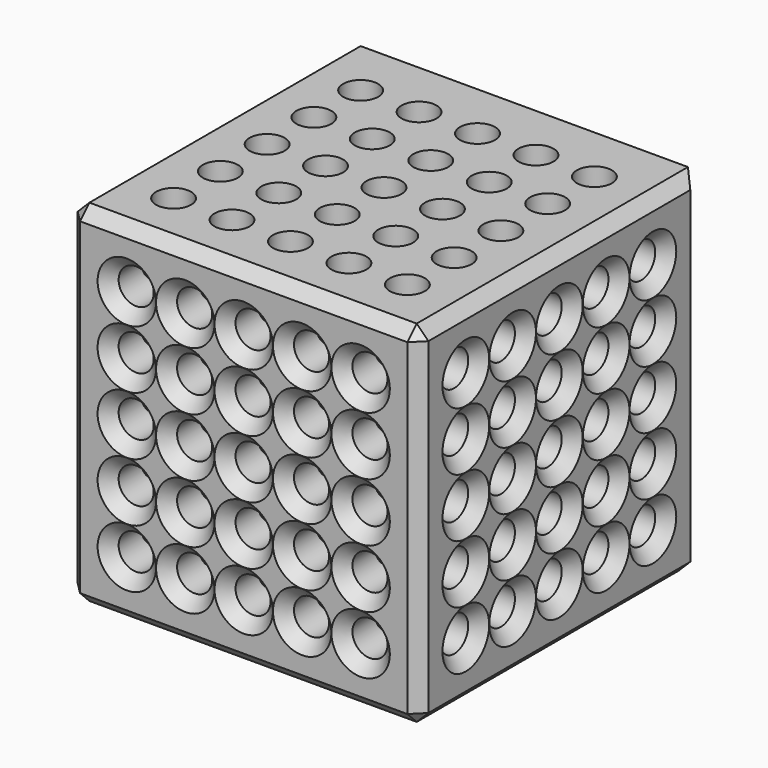
from build123d import *

# Parameters (mm, degrees)
F0_W     = 150
F0_H     = 150
F1_DEPTH = 150
F2_R     = 7.5
F3_DEPTH = 150.001
F4_R     = 7.5
F5_DEPTH = 150.001
F6_R     = 7.5
F7_DEPTH = 150.001
F8_SIZE  = 4.99999


# Not quite as in the source:
# - a fillet or chamfer is up to 0.001 mm smaller than in the source, because OpenCascade refuses the exact size


with BuildPart() as f1:
    # F0 (on Front) → F1 (new body)
    with BuildSketch(Plane.XZ):
        Rectangle(F0_W, F0_H)
    extrude(amount=F1_DEPTH)

    # F2 (on face) → F3 (cut, through all)
    with BuildSketch(Plane.XZ.offset(150)):
        with Locations((50, 50)):
            Circle(F2_R)
        with Locations((50, 25)):
            Circle(F2_R)
        with Locations((50, 0)):
            Circle(F2_R)
        with Locations((50, -25)):
            Circle(F2_R)
        with Locations((50, -50)):
            Circle(F2_R)
        with Locations((25, 50)):
            Circle(F2_R)
        with Locations((25, 25)):
            Circle(F2_R)
        with Locations((25, 0)):
            Circle(F2_R)
        with Locations((25, -25)):
            Circle(F2_R)
        with Locations((25, -50)):
            Circle(F2_R)
        with Locations((0, 50)):
            Circle(F2_R)
        with Locations((0, 25)):
            Circle(F2_R)
        Circle(F2_R)
        with Locations((0, -25)):
            Circle(F2_R)
        with Locations((0, -50)):
            Circle(F2_R)
        with Locations((-25, 50)):
            Circle(F2_R)
        with Locations((-25, 25)):
            Circle(F2_R)
        with Locations((-25, 0)):
            Circle(F2_R)
        with Locations((-25, -25)):
            Circle(F2_R)
        with Locations((-25, -50)):
            Circle(F2_R)
        with Locations((-50, 50)):
            Circle(F2_R)
        with Locations((-50, 25)):
            Circle(F2_R)
        with Locations((-50, 0)):
            Circle(F2_R)
        with Locations((-50, -25)):
            Circle(F2_R)
        with Locations((-50, -50)):
            Circle(F2_R)
    extrude(amount=-F3_DEPTH, mode=Mode.SUBTRACT)

    # F4 (on face) → F5 (cut, through all)
    with BuildSketch(Plane.YZ.offset(75)):
        with Locations((-25, 50)):
            Circle(F4_R)
        with Locations((-25, 25)):
            Circle(F4_R)
        with Locations((-25, 0)):
            Circle(F4_R)
        with Locations((-25, -25)):
            Circle(F4_R)
        with Locations((-25, -50)):
            Circle(F4_R)
        with Locations((-50, 50)):
            Circle(F4_R)
        with Locations((-50, 25)):
            Circle(F4_R)
        with Locations((-50, 0)):
            Circle(F4_R)
        with Locations((-50, -25)):
            Circle(F4_R)
        with Locations((-50, -50)):
            Circle(F4_R)
        with Locations((-75, 50)):
            Circle(F4_R)
        with Locations((-75, 25)):
            Circle(F4_R)
        with Locations((-75, 0)):
            Circle(F4_R)
        with Locations((-75, -25)):
            Circle(F4_R)
        with Locations((-75, -50)):
            Circle(F4_R)
        with Locations((-100, 50)):
            Circle(F4_R)
        with Locations((-100, 25)):
            Circle(F4_R)
        with Locations((-100, 0)):
            Circle(F4_R)
        with Locations((-100, -25)):
            Circle(F4_R)
        with Locations((-100, -50)):
            Circle(F4_R)
        with Locations((-125, 50)):
            Circle(F4_R)
        with Locations((-125, 25)):
            Circle(F4_R)
        with Locations((-125, 0)):
            Circle(F4_R)
        with Locations((-125, -25)):
            Circle(F4_R)
        with Locations((-125, -50)):
            Circle(F4_R)
    extrude(amount=-F5_DEPTH, mode=Mode.SUBTRACT)

    # F6 (on face) → F7 (cut, through all)
    with BuildSketch(Plane(origin=(0, 0, -75), x_dir=(1, 0, 0), z_dir=(0, 0, -1))):
        with Locations((50, 125)):
            Circle(F6_R)
        with Locations((50, 100)):
            Circle(F6_R)
        with Locations((50, 75)):
            Circle(F6_R)
        with Locations((50, 50)):
            Circle(F6_R)
        with Locations((50, 25)):
            Circle(F6_R)
        with Locations((25, 125)):
            Circle(F6_R)
        with Locations((25, 100)):
            Circle(F6_R)
        with Locations((25, 75)):
            Circle(F6_R)
        with Locations((25, 50)):
            Circle(F6_R)
        with Locations((25, 25)):
            Circle(F6_R)
        with Locations((0, 125)):
            Circle(F6_R)
        with Locations((0, 100)):
            Circle(F6_R)
        with Locations((0, 75)):
            Circle(F6_R)
        with Locations((0, 50)):
            Circle(F6_R)
        with Locations((0, 25)):
            Circle(F6_R)
        with Locations((-25, 125)):
            Circle(F6_R)
        with Locations((-25, 100)):
            Circle(F6_R)
        with Locations((-25, 75)):
            Circle(F6_R)
        with Locations((-25, 50)):
            Circle(F6_R)
        with Locations((-25, 25)):
            Circle(F6_R)
        with Locations((-50, 125)):
            Circle(F6_R)
        with Locations((-50, 100)):
            Circle(F6_R)
        with Locations((-50, 75)):
            Circle(F6_R)
        with Locations((-50, 50)):
            Circle(F6_R)
        with Locations((-50, 25)):
            Circle(F6_R)
    extrude(amount=-F7_DEPTH, mode=Mode.SUBTRACT)

    # F8 (size 5 in the source; OpenCascade refuses exactly that, so slightly less here)
    f8_edges = [f1.edges().sort_by_distance(p)[0] for p in [
        (-75, -75, 75),
        (-75, 0, 0),
        (-75, -150, 0),
        (-75, -75, -75),
        (-75, -132.5, 50),
        (-75, -132.5, 25),
        (-75, -107.5, 50),
        (-75, -107.5, 25),
        (-75, -132.5, 0),
        (-75, -132.5, -25),
        (-75, -132.5, -50),
        (-75, -107.5, 0),
        (-75, -107.5, -25),
        (-75, -107.5, -50),
        (-75, -82.5, 50),
        (-75, -57.5, 50),
        (-75, -82.5, 25),
        (-75, -57.5, 25),
        (-75, -32.5, 50),
        (-75, -32.5, 25),
        (-75, -82.5, 0),
        (-75, -82.5, -25),
        (-75, -57.5, 0),
        (-75, -57.5, -25),
        (-75, -82.5, -50),
        (-75, -57.5, -50),
        (-75, -32.5, 0),
        (-75, -32.5, -25),
        (-75, -32.5, -50),
        (0, 0, -75),
        (0, -150, -75),
        (75, -75, -75),
        (-57.5, -125, -75),
        (-32.5, -125, -75),
        (-57.5, -100, -75),
        (-32.5, -100, -75),
        (-7.5, -125, -75),
        (17.5, -125, -75),
        (42.5, -125, -75),
        (-7.5, -100, -75),
        (17.5, -100, -75),
        (42.5, -100, -75),
        (-57.5, -75, -75),
        (-57.5, -50, -75),
        (-32.5, -75, -75),
        (-32.5, -50, -75),
        (-57.5, -25, -75),
        (-32.5, -25, -75),
        (-7.5, -75, -75),
        (17.5, -75, -75),
        (-7.5, -50, -75),
        (17.5, -50, -75),
        (42.5, -75, -75),
        (42.5, -50, -75),
        (-7.5, -25, -75),
        (17.5, -25, -75),
        (42.5, -25, -75),
        (75, 0, 0),
        (75, -150, 0),
        (75, -75, 75),
        (75, -132.5, -50),
        (75, -132.5, -25),
        (75, -107.5, -50),
        (75, -107.5, -25),
        (75, -132.5, 0),
        (75, -132.5, 25),
        (75, -132.5, 50),
        (75, -107.5, 0),
        (75, -107.5, 25),
        (75, -107.5, 50),
        (75, -82.5, -50),
        (75, -57.5, -50),
        (75, -82.5, -25),
        (75, -57.5, -25),
        (75, -32.5, -50),
        (75, -32.5, -25),
        (75, -82.5, 0),
        (75, -82.5, 25),
        (75, -57.5, 0),
        (75, -57.5, 25),
        (75, -82.5, 50),
        (75, -57.5, 50),
        (75, -32.5, 0),
        (75, -32.5, 25),
        (75, -32.5, 50),
        (0, -150, 75),
        (-57.5, -150, -50),
        (-32.5, -150, -50),
        (-57.5, -150, -25),
        (-32.5, -150, -25),
        (-7.5, -150, -50),
        (17.5, -150, -50),
        (42.5, -150, -50),
        (-7.5, -150, -25),
        (17.5, -150, -25),
        (42.5, -150, -25),
        (-57.5, -150, 0),
        (-57.5, -150, 25),
        (-32.5, -150, 0),
        (-32.5, -150, 25),
        (-57.5, -150, 50),
        (-32.5, -150, 50),
        (-7.5, -150, 0),
        (17.5, -150, 0),
        (-7.5, -150, 25),
        (17.5, -150, 25),
        (42.5, -150, 0),
        (42.5, -150, 25),
        (-7.5, -150, 50),
        (17.5, -150, 50),
        (42.5, -150, 50),
    ]]
    chamfer(f8_edges, length=F8_SIZE)


solid = f1.part
